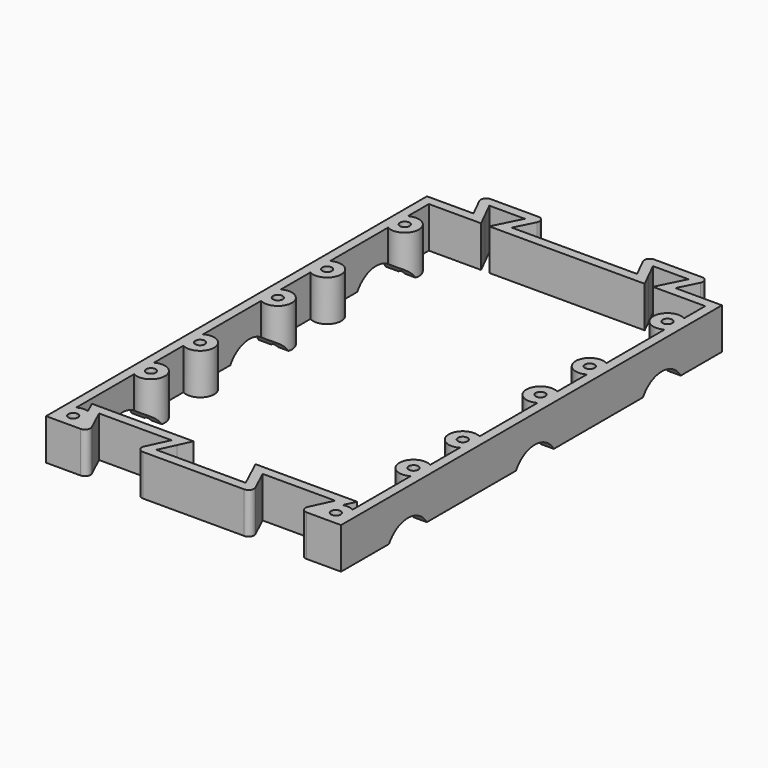
from build123d import *

# Parameters (mm, degrees)
F0_R        = 1.75
F1_DEPTH    = 15
F2_T        = 3.4
F2_T3_DEPTH = 21.8
F3_R        = 2
F5_DEPTH    = 200


# Not quite as in the source:
# - a shell that OpenCascade refuses in one call is made with other operations: the cavity is built on its own and cut out


with BuildPart() as f1:
    # F0 (on Top) → F1 (new body)
    with BuildSketch(Plane.XY):
        Polygon((17, 0), (0, 0), (0, -174), (15.75, -174), (10.75, -163.25), (37.25, -163.25), (32.25, -174), (75.55, -174), (70.55, -163.25), (97.05, -163.25), (92.05, -174), (107.8, -174), (107.8, 0), (90.8, 0), (95.8, 10), (71.8, 10), (76.8, 0), (31, 0), (36, 10), (12, 10), align=None)
        with Locations((5.9, -169)):
            Circle(F0_R, mode=Mode.SUBTRACT)
        with Locations((5.9, -133.5)):
            Circle(F0_R, mode=Mode.SUBTRACT)
        with Locations((5.9, -111)):
            Circle(F0_R, mode=Mode.SUBTRACT)
        with Locations((5.9, -75.5)):
            Circle(F0_R, mode=Mode.SUBTRACT)
        with Locations((101.9, -169)):
            Circle(F0_R, mode=Mode.SUBTRACT)
        with Locations((101.9, -133.5)):
            Circle(F0_R, mode=Mode.SUBTRACT)
        with Locations((101.9, -111)):
            Circle(F0_R, mode=Mode.SUBTRACT)
        with Locations((101.9, -75.5)):
            Circle(F0_R, mode=Mode.SUBTRACT)
        with Locations((5.9, -53)):
            Circle(F0_R, mode=Mode.SUBTRACT)
        with Locations((5.9, -17.5)):
            Circle(F0_R, mode=Mode.SUBTRACT)
        with Locations((101.9, -53)):
            Circle(F0_R, mode=Mode.SUBTRACT)
        with Locations((101.9, -17.5)):
            Circle(F0_R, mode=Mode.SUBTRACT)
    extrude(amount=F1_DEPTH)

    # F2: shell of thickness 3.4, made by hand


with BuildPart() as f2_core1:
    # F2_t2: copy of F1
    add(f1.part)

    # the walls: a layer under each face that stays
    f2_faces = [f2_core1.faces().sort_by_distance(p)[0] for p in [
        (8.5, 0, 7.5),
        (0, -87, 7.5),
        (7.875, -174, 7.5),
        (13.25, -168.625, 7.5),
        (24, -163.25, 7.5),
        (34.75, -168.625, 7.5),
        (53.9, -174, 7.5),
        (73.05, -168.625, 7.5),
        (83.8, -163.25, 7.5),
        (94.55, -168.625, 7.5),
        (99.925, -174, 7.5),
        (107.8, -87, 7.5),
        (99.3, 0, 7.5),
        (93.3, 5, 7.5),
        (83.8, 10, 7.5),
        (74.3, 5, 7.5),
        (53.9, 0, 7.5),
        (33.5, 5, 7.5),
        (24, 10, 7.5),
        (14.5, 5, 7.5),
        (4.15, -169, 7.5),
        (4.15, -133.5, 7.5),
        (4.15, -111, 7.5),
        (4.15, -75.5, 7.5),
        (100.15, -169, 7.5),
        (100.15, -133.5, 7.5),
        (100.15, -111, 7.5),
        (100.15, -75.5, 7.5),
        (4.15, -53, 7.5),
        (4.15, -17.5, 7.5),
        (100.15, -53, 7.5),
        (100.15, -17.5, 7.5),
    ]]
    thicken(f2_faces, amount=-F2_T, mode=Mode.SUBTRACT)

    # F2_s4 → F2_t3 (cut)
    with BuildSketch(Plane.XY.offset(-3.4)):
        Polygon((16.9695894755, 0.0187947378), (17, -3.4), (22.5013155617, -3.4), (20.0410524494, 1.5205262247), align=None)
        Polygon((10.7808285178, -163.2696611545), (7.6671482196, -164.683884549), (5.4188298247, -159.85), (10.75, -159.85), align=None)
        Polygon((37.2191714822, -163.2696611545), (37.25, -159.85), (42.5811701753, -159.85), (40.3328517804, -164.683884549), align=None)
        Polygon((70.5808285178, -163.2696611545), (67.4671482196, -164.683884549), (65.2188298247, -159.85), (70.55, -159.85), align=None)
        Polygon((97.0191714822, -163.2696611545), (97.05, -159.85), (102.3811701753, -159.85), (100.1328517804, -164.683884549), align=None)
        Polygon((90.8304105245, 0.0187947378), (90.8, -3.4), (85.2986844383, -3.4), (87.7589475506, 1.5205262247), align=None)
        Polygon((76.7695894755, 0.0187947378), (79.8410524494, 1.5205262247), (82.3013155617, -3.4), (76.8, -3.4), align=None)
        Polygon((31.0304105245, 0.0187947378), (31, -3.4), (25.4986844383, -3.4), (27.9589475506, 1.5205262247), align=None)
    extrude(amount=F2_T3_DEPTH, mode=Mode.SUBTRACT)


with BuildPart() as f1_1:
    add(f1.part)

    # what is left inside the walls is the cavity
    f2_cavity = [f2_core1.part.solids().sort_by_distance(p)[0] for p in [
        (53.9, -111.533333, 14.966),
    ]]
    add(f2_cavity, mode=Mode.SUBTRACT)

    # F3
    f3_edges = [f1_1.edges().sort_by_distance(p)[0] for p in [
        (15.75, -174, 7.5),
        (32.25, -174, 7.5),
        (75.55, -174, 7.5),
        (92.05, -174, 7.5),
        (12, 10, 7.5),
        (36, 10, 7.5),
        (71.8, 10, 7.5),
        (95.8, 10, 7.5),
    ]]
    fillet(f3_edges, radius=F3_R)

    # F4 (on face) → F5 (cut)
    with BuildSketch(Plane.YZ.offset(107.8)):
        with BuildLine():
            Line((-152.0961523056, 0), (-134.8088085651, 0))
            ThreePointArc((-134.8088085651, 0), (-143.4524804354, 4.8799020536), (-152.0961523056, 0))
        make_face()
        with BuildLine():
            ThreePointArc((-76.8088085651, 0), (-85.4524804354, 4.8799020536), (-94.0961523056, 0))
            Line((-94.0961523056, 0), (-76.8088085651, 0))
        make_face()
        with BuildLine():
            ThreePointArc((-18.8088085651, 0), (-27.4524804354, 4.8799020536), (-36.0961523056, 0))
            Line((-36.0961523056, 0), (-18.8088085651, 0))
        make_face()
    extrude(amount=-F5_DEPTH, mode=Mode.SUBTRACT)


solid = f1_1.part
